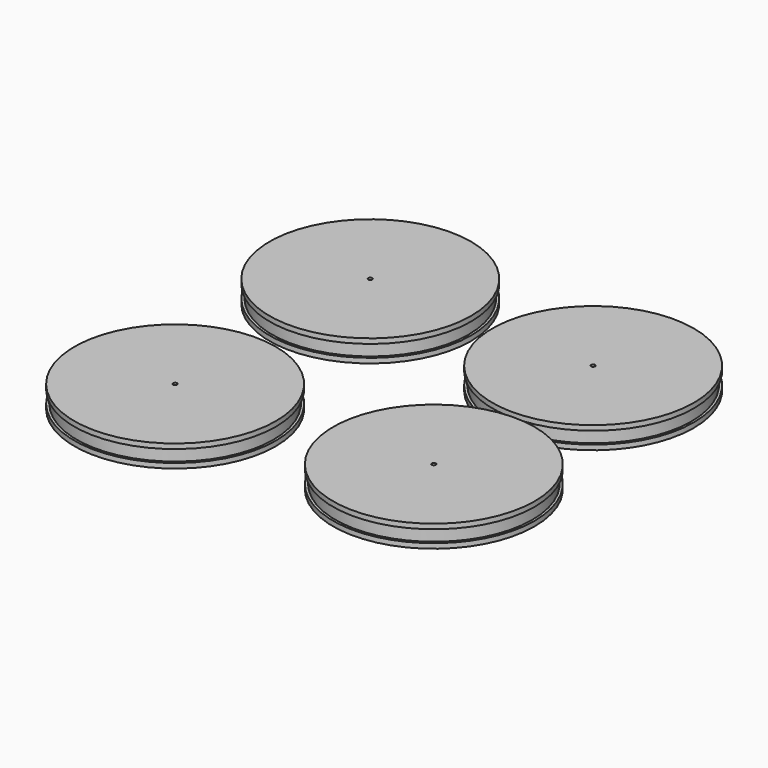
from build123d import *

# Parameters (mm, degrees)
F0_R      = 40
F1_DEPTH  = 5
F2_R      = 0.835
F3_DEPTH  = 5.001
F3_TAPER  = -4
F4_R      = 0.835
F5_DEPTH  = 5.0010001
F5_TAPER  = -4
F6_R      = 0.835
F7_DEPTH  = 5.0010001
F7_TAPER  = -4
F8_R      = 0.835
F9_DEPTH  = 5.0010001
F9_TAPER  = -4
F13_R     = 41
F14_DEPTH = 2
F12_R     = 41
F11_R     = 41
F10_R     = 41
F15_R     = 41
F19_DEPTH = 2
F16_R     = 41
F17_R     = 41
F18_R     = 41
F20_R     = 0.835
F21_R     = 0.835
F22_R     = 0.835
F23_R     = 0.835
F24_DEPTH = 9.001


with BuildPart() as f1:
    # F0 (on Top) → F1 (new body)
    with BuildSketch(Plane.XY):
        with Locations((-43.1832037866, 36.8267968297)):
            Circle(F0_R)
    extrude(amount=F1_DEPTH)

    # F2 (on face) → F3 (cut, through all)
    with BuildSketch(Plane.XY.offset(5)):
        with Locations((-43.1832037866, 36.8267968297)):
            Circle(F2_R)
    extrude(amount=-F3_DEPTH, taper=F3_TAPER, mode=Mode.SUBTRACT)

    # F10 (on face) → F14, piece 4 (join)
    with BuildSketch(Plane.XY.offset(5)):
        with Locations((-43.1832037866, 36.8267968297)):
            Circle(F10_R)
    extrude(amount=F14_DEPTH)


with BuildPart() as f1b:
    # F0 (on Top) → F1, piece 2 (new body)
    with BuildSketch(Plane.XY):
        with Locations((49.4387149811, 34.4053097069)):
            Circle(F0_R)
    extrude(amount=F1_DEPTH)

    # F4 (on face) → F5 (cut, through all)
    with BuildSketch(Plane.XY.offset(5)):
        with Locations((49.4387149811, 34.4053097069)):
            Circle(F4_R)
    extrude(amount=-F5_DEPTH, taper=F5_TAPER, mode=Mode.SUBTRACT)

    # F11 (on face) → F14, piece 3 (join)
    with BuildSketch(Plane.XY.offset(5)):
        with Locations((49.4387149811, 34.4053097069)):
            Circle(F11_R)
    extrude(amount=F14_DEPTH)


with BuildPart() as f1c:
    # F0 (on Top) → F1, piece 3 (new body)
    with BuildSketch(Plane.XY):
        with Locations((-46.4118532836, -58.4184005857)):
            Circle(F0_R)
    extrude(amount=F1_DEPTH)

    # F6 (on face) → F7 (cut, through all)
    with BuildSketch(Plane.XY.offset(5)):
        with Locations((-46.4118532836, -58.4184005857)):
            Circle(F6_R)
    extrude(amount=-F7_DEPTH, taper=F7_TAPER, mode=Mode.SUBTRACT)

    # F12 (on face) → F14, piece 2 (join)
    with BuildSketch(Plane.XY.offset(5)):
        with Locations((-46.4118532836, -58.4184005857)):
            Circle(F12_R)
    extrude(amount=F14_DEPTH)

    # F15 (on face) → F19 (join)
    with BuildSketch(Plane(origin=(0, 0, 0), x_dir=(1, 0, 0), z_dir=(0, 0, -1))):
        with Locations((-46.4118532836, 58.4184005857)):
            Circle(F15_R)
    extrude(amount=F19_DEPTH)


with BuildPart() as f1d:
    # F0 (on Top) → F1, piece 4 (new body)
    with BuildSketch(Plane.XY):
        with Locations((52.2637851536, -50.1449815929)):
            Circle(F0_R)
    extrude(amount=F1_DEPTH)

    # F8 (on face) → F9 (cut, through all)
    with BuildSketch(Plane.XY.offset(5)):
        with Locations((52.2637851536, -50.1449815929)):
            Circle(F8_R)
    extrude(amount=-F9_DEPTH, taper=F9_TAPER, mode=Mode.SUBTRACT)

    # F13 (on face) → F14 (join)
    with BuildSketch(Plane.XY.offset(5)):
        with Locations((52.2637851536, -50.1449815929)):
            Circle(F13_R)
    extrude(amount=F14_DEPTH)


with BuildPart() as f19:
    # F16 (on face) → F19, piece 2 (new body)
    with BuildSketch(Plane(origin=(0, 0, 0), x_dir=(1, 0, 0), z_dir=(0, 0, -1))):
        with Locations((52.2637851536, 50.1449815929)):
            Circle(F16_R)
    extrude(amount=F19_DEPTH)


with BuildPart() as f19b:
    # F17 (on face) → F19, piece 3 (new body)
    with BuildSketch(Plane(origin=(0, 0, 0), x_dir=(1, 0, 0), z_dir=(0, 0, -1))):
        with Locations((-43.1832037866, -36.8267968297)):
            Circle(F17_R)
    extrude(amount=F19_DEPTH)


with BuildPart() as f19c:
    # F18 (on face) → F19, piece 4 (new body)
    with BuildSketch(Plane(origin=(0, 0, 0), x_dir=(1, 0, 0), z_dir=(0, 0, -1))):
        with Locations((49.4387149811, -34.4053097069)):
            Circle(F18_R)
    extrude(amount=F19_DEPTH)


with BuildPart() as f24_tool:
    # F20 (on face) + F21 (on face) + F22 (on face) + F23 (on face) → F24 (new body, through all)
    with BuildSketch(Plane.XY.offset(7)):
        with Locations((-43.1832037866, 36.8267968297)):
            Circle(F20_R)
    with BuildSketch(Plane.XY.offset(7)):
        with Locations((-46.4118532836, -58.4184005857)):
            Circle(F21_R)
    with BuildSketch(Plane.XY.offset(7)):
        with Locations((52.2637851536, -50.1449815929)):
            Circle(F22_R)
    with BuildSketch(Plane.XY.offset(7)):
        with Locations((49.4387149811, 34.4053097069)):
            Circle(F23_R)
    extrude(amount=-F24_DEPTH)


with BuildPart() as f1_1:
    add(f1.part)

    # F24: cut by f24_tool
    add(f24_tool.part, mode=Mode.SUBTRACT)


with BuildPart() as f1b_1:
    add(f1b.part)

    # F24: cut by f24_tool
    add(f24_tool.part, mode=Mode.SUBTRACT)


with BuildPart() as f1c_1:
    add(f1c.part)

    # F24: cut by f24_tool
    add(f24_tool.part, mode=Mode.SUBTRACT)


with BuildPart() as f1d_1:
    add(f1d.part)

    # F24: cut by f24_tool
    add(f24_tool.part, mode=Mode.SUBTRACT)


with BuildPart() as f19_1:
    add(f19.part)

    # F24: cut by f24_tool
    add(f24_tool.part, mode=Mode.SUBTRACT)


with BuildPart() as f19b_1:
    add(f19b.part)

    # F24: cut by f24_tool
    add(f24_tool.part, mode=Mode.SUBTRACT)


with BuildPart() as f19c_1:
    add(f19c.part)

    # F24: cut by f24_tool
    add(f24_tool.part, mode=Mode.SUBTRACT)


solid = Compound([f1_1.part, f1b_1.part, f1c_1.part, f1d_1.part, f19_1.part, f19b_1.part, f19c_1.part])
